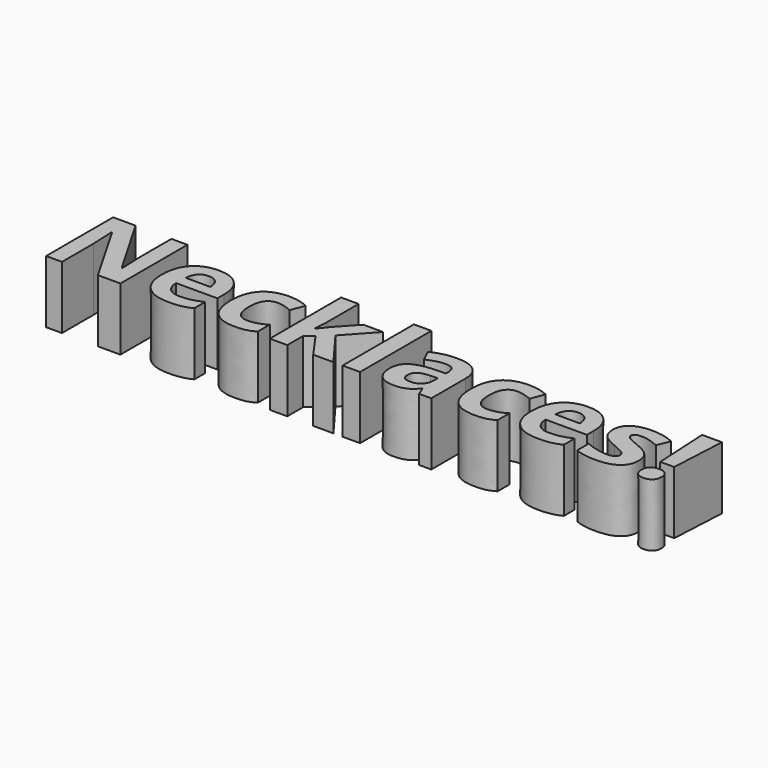
from build123d import *

# Parameters (mm, degrees)
F0_TEXT_SIZE = 9.5092132202
F1_DEPTH     = 5.08


# Not quite as in the source:
# - Text() gives the source's letters only with a copy of the font that has no kerning and outlines rounded to 1/6400 em; it was checked with that copy


with BuildPart() as f1:
    # F0 (on Top) → F1 (new body)
    with BuildSketch(Plane.XY):
        with Locations((-26.2334148115, -2.8467577706)):
            Text('Necklaces!', F0_TEXT_SIZE, font='Open Sans', font_style=FontStyle.BOLD, text_align=(TextAlign.LEFT, TextAlign.BOTTOM))
    extrude(amount=F1_DEPTH)


solid = f1.part
